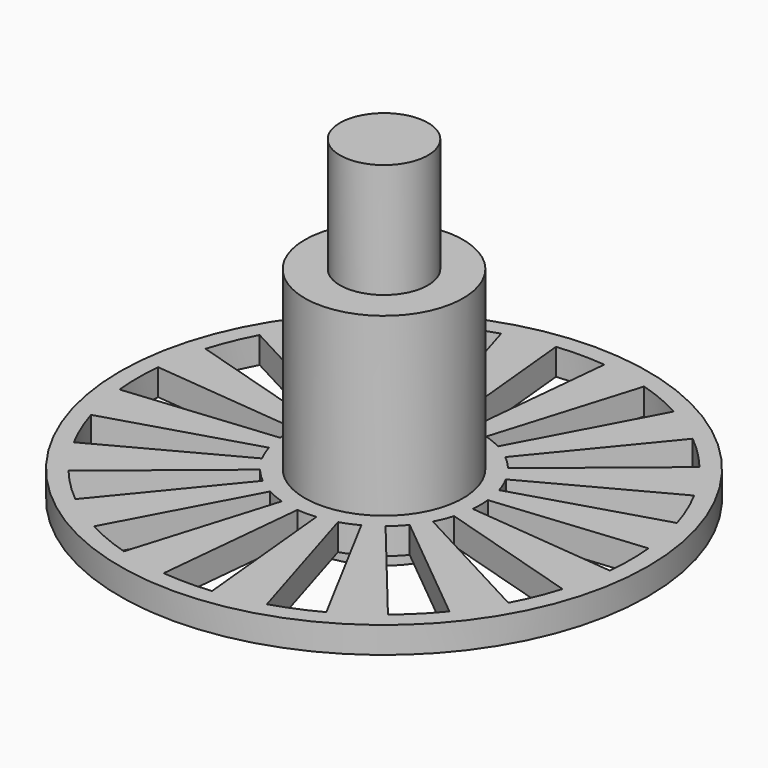
from build123d import *

# Parameters (mm, degrees)
F3_D            = 2.5
F3_DEPTH        = 6.5
F3_TIP          = 0.7510757738
F5_DEPTH        = 2.501
F5_COPIES_COUNT = 16


# Not quite as in the source:
# - a pattern or mirror of a feature is missing from the dataset's text; its kind, count and spacing are read off the source's solid


with BuildPart() as f1:
    # F0 (on Front) → F1 (revolve)
    with BuildSketch(Plane.XZ):
        Polygon((-4.5, 0), (-3, 0), (-3, 7.5), (0, 7.5), (0, 19), (-2.5, 19), (-2.5, 12.5), (-4.5, 12.5), (-4.5, 2.5), (-15, 2.5), (-15, 1), (-4.5, 1), align=None)
    revolve(axis=Axis((0, 0, 13.1862424314), (0, 0, 1)))

    # F3
    with Locations(Plane(origin=(0, 0, 7.5), x_dir=(1, 0, 0), z_dir=(0, 0, -1))):
        with Locations((0, 0)):
            Hole(F3_D / 2, depth=F3_DEPTH)
            with Locations((0, 0, -(F3_DEPTH + F3_TIP / 2))):  # 118° drill point
                Cone(0, F3_D / 2, F3_TIP, mode=Mode.SUBTRACT)

    # F4 (on face) → F5 (cut, through all)
    with BuildSketch(Plane.XY.offset(2.5)):
        with BuildLine():
            Line((-1.3722399646, 13.9325861734), (-0.5390942718, 5.4735159967))
            ThreePointArc((-0.5390942718, 5.4735159967), (0, 5.5), (0.5390942718, 5.4735159967))
            Line((0.5390942718, 5.4735159967), (1.3722399646, 13.9325861734))
            ThreePointArc((1.3722399646, 13.9325861734), (0, 14), (-1.3722399646, 13.9325861734))
        make_face()
    f5 = extrude(amount=-F5_DEPTH, mode=Mode.SUBTRACT)

    # F5_copies: F5 ×16 about axis
    f5_copies_axis = Axis((0, 0, 0), (0, 0, 1))
    for i in range(1, F5_COPIES_COUNT):
        add(f5.rotate(f5_copies_axis, i * 360 / F5_COPIES_COUNT), mode=Mode.SUBTRACT)


solid = f1.part
